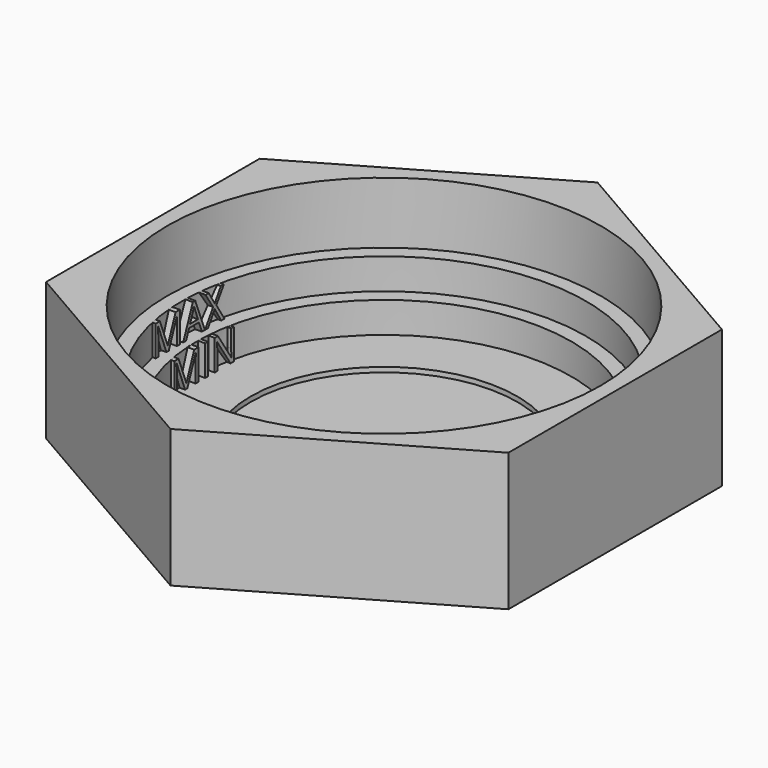
from build123d import *

# Parameters (mm, degrees)
F0_R          = 27.5
F1_DEPTH      = 2
F2_DEPTH      = 3
F3_R          = 44.6313972081
F4_DEPTH      = 25.4
F5_R          = 44.6313972081
F5_R_2        = 41.6313972081
F6_DEPTH      = 12.7
F7_R          = 41.6313972081
F7_R_2        = 38.6313972081
F8_DEPTH      = 6.35
F10_START     = -37.2
F9_TEXT_SIZE  = 8.8194444444
F10_DEPTH     = 3.4
F12_START     = -40.08
F11_TEXT_SIZE = 8.8194444444
F12_DEPTH     = 5.42


# Not quite as in the source:
# - a length typed as a fraction of an inch, garbled in the dataset ("3 / 203.2 mm" for 3/8 in), is restored
# - Text() gives the source's letters only with a copy of the font that has no kerning and outlines rounded to 1/6400 em; it was checked with that copy


with BuildPart() as f1:
    # F0 (on Top) → F1 (new body)
    with BuildSketch(Plane.XY):
        Polygon((0, -55), (47.6313972081, -27.5), (47.6313972081, 27.5), (0, 55), (-47.6313972081, 27.5), (-47.6313972081, -27.5), align=None)
        Circle(F0_R, mode=Mode.SUBTRACT)
        Circle(F0_R)
    extrude(amount=F1_DEPTH)

    # F0 (on Top) → F2 (join)
    with BuildSketch(Plane.XY):
        Polygon((0, -55), (47.6313972081, -27.5), (47.6313972081, 27.5), (0, 55), (-47.6313972081, 27.5), (-47.6313972081, -27.5), align=None)
        Circle(F0_R, mode=Mode.SUBTRACT)
    extrude(amount=F2_DEPTH)

    # F3 (on face) → F4 (join)
    with BuildSketch(Plane.XY.offset(3)):
        Polygon((-47.6313972081, 27.5), (-47.6313972081, -27.5), (0, -55), (47.6313972081, -27.5), (47.6313972081, 27.5), (0, 55), align=None)
        Circle(F3_R, mode=Mode.SUBTRACT)
    extrude(amount=F4_DEPTH)

    # F5 (on face) → F6 (join)
    with BuildSketch(Plane.XY.offset(3)):
        Circle(F5_R)
        Circle(F5_R_2, mode=Mode.SUBTRACT)
    extrude(amount=F6_DEPTH)

    # F7 (on face) → F8 (join)
    with BuildSketch(Plane.XY.offset(3)):
        Circle(F7_R)
        Circle(F7_R_2, mode=Mode.SUBTRACT)
    extrude(amount=F8_DEPTH)

    # F9 (on Right) → F10 (join)
    with BuildSketch(Plane.YZ.offset(F10_START)):
        with Locations((-8.3881184896, 3)):
            Text('MIN', F9_TEXT_SIZE, font='Open Sans', text_align=(TextAlign.LEFT, TextAlign.BOTTOM))
    extrude(amount=-F10_DEPTH)

    # F11 (on Right) → F12 (join)
    with BuildSketch(Plane.YZ.offset(F12_START)):
        with Locations((-9.5856336806, 9.35)):
            Text('MAX', F11_TEXT_SIZE, font='Open Sans', text_align=(TextAlign.LEFT, TextAlign.BOTTOM))
    extrude(amount=-F12_DEPTH)


solid = f1.part
